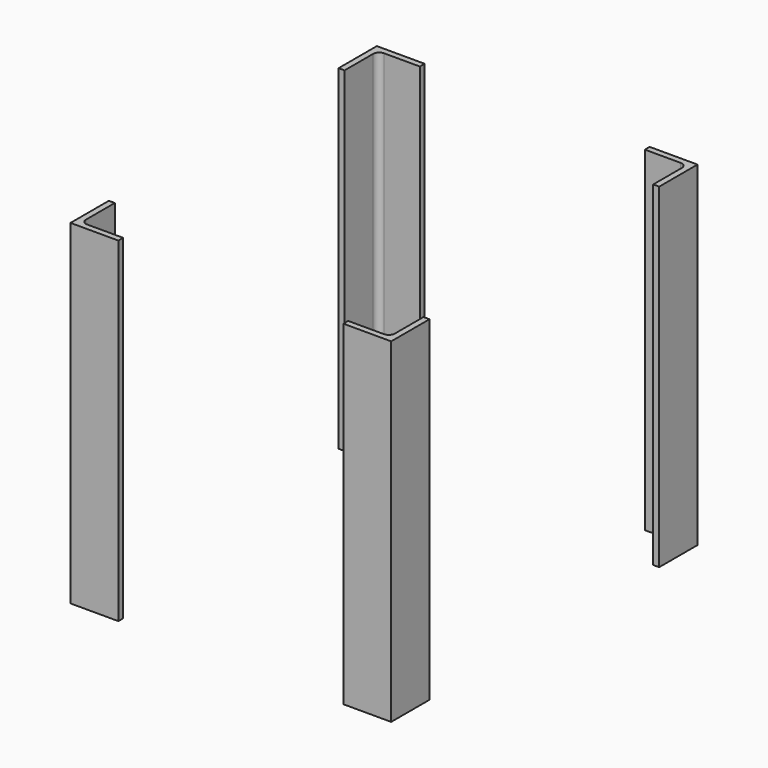
from build123d import *

# Parameters (mm, degrees)
F1_DEPTH = 177.8
F4_R     = 3.175


# Not quite as in the source:
# - a length typed as a fraction of an inch, garbled in the dataset ("3 / 203.2 mm" for 3/8 in), is restored


with BuildPart() as f1:
    # F0 (on Top) → F1 (new body)
    with BuildSketch(Plane.XY):
        Polygon((25.4, 0), (0, 0), (0, -25.4), (3.175, -25.4), (3.175, -3.175), (25.4, -3.175), align=None)
    extrude(amount=F1_DEPTH)

    # F4
    f4_edges = [f1.edges().sort_by_distance(p)[0] for p in [
        (3.175, -3.175, 88.9),
    ]]
    fillet(f4_edges, radius=F4_R)


with BuildPart() as f5_1:
    # F5: instance of F1
    add(f1.part.mirror(Plane.XZ.offset(101.6)))


with BuildPart() as f6_1:
    # F6: instance of F1
    add(f1.part.mirror(Plane.YZ.offset(85.09)))


with BuildPart() as f6_2:
    # F6: instance of F5_1
    add(f5_1.part.mirror(Plane.YZ.offset(85.09)))


solid = Compound([f1.part, f5_1.part, f6_1.part, f6_2.part])
